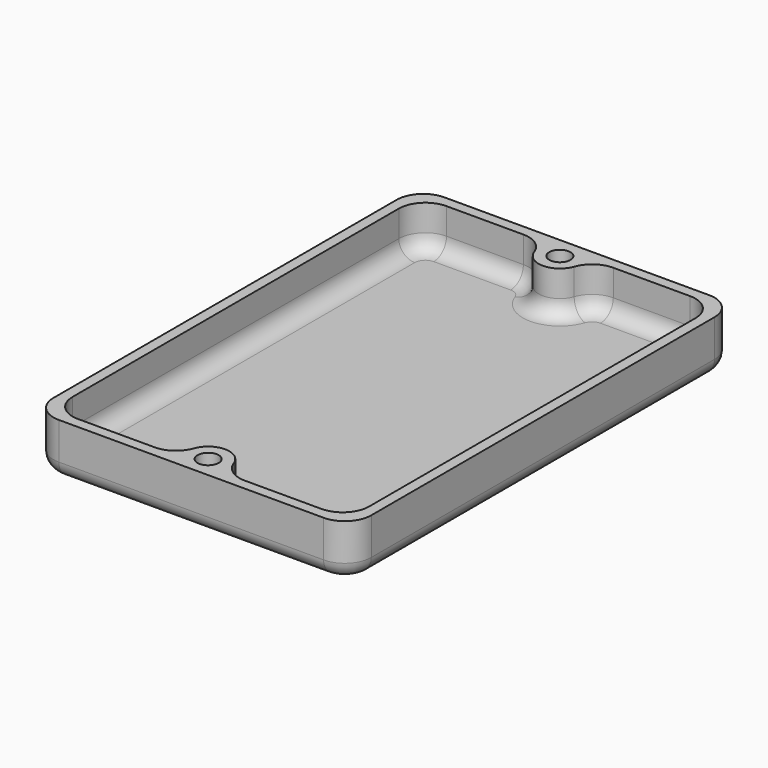
from build123d import *

# Parameters (mm, degrees)
F3_W          = 60
F3_H          = 91
F4_DEPTH      = 10
F5_W          = 56
F5_H          = 87
F6_DEPTH      = 8
F7_R          = 4
F8_DEPTH      = 10
F9_R          = 2
F10_DEPTH     = 10.001
F11_R         = 5
F12_R         = 5
F13_T1_DEPTH  = 77
F13_T3_DEPTH  = 14.5147186258
F13_T5_DEPTH  = 14.5147186258
F13_T8_ANGLE  = 90
F13_T10_ANGLE = 70.5287793655
F13_T12_ANGLE = 141.057558731
F13_T14_ANGLE = 90
F13_T16_ANGLE = 70.5287793655
F13_T18_ANGLE = 70.5287793655
F13_T20_ANGLE = 90
F13_T22_ANGLE = 141.057558731
F13_T24_ANGLE = 70.5287793655
F13_T26_ANGLE = 90
F13_T27_DEPTH = 81
F13_T29_DEPTH = 50
F13_T32_ANGLE = 90
F13_T34_ANGLE = 90
F13_T36_ANGLE = 90
F13_T38_ANGLE = 90


# Not quite as in the source:
# - a fillet or chamfer that OpenCascade refuses, or shapes differently, is made with other operations: its cross-section is extruded or revolved along the edge and cut away or added


with BuildPart() as f4:
    # F3 (on Top) → F4 (new body)
    with BuildSketch(Plane.XY):
        Rectangle(F3_W, F3_H)
    extrude(amount=F4_DEPTH)

    # F5 (on face) → F6 (cut)
    with BuildSketch(Plane.XY.offset(10)):
        Rectangle(F5_W, F5_H)
    extrude(amount=-F6_DEPTH, mode=Mode.SUBTRACT)

    # F7 (on face) → F8 (join)
    with BuildSketch(Plane(origin=(0, 0, 0), x_dir=(1, 0, 0), z_dir=(0, 0, -1))):
        with Locations((0, -41.5)):
            Circle(F7_R)
        with Locations((0, 41.5)):
            Circle(F7_R)
    extrude(amount=-F8_DEPTH)

    # F9 (on face) → F10 (cut, through all)
    with BuildSketch(Plane(origin=(0, 0, 0), x_dir=(1, 0, 0), z_dir=(0, 0, -1))):
        with Locations((0, -41.5)):
            Circle(F9_R)
        with Locations((0, 41.5)):
            Circle(F9_R)
    extrude(amount=-F10_DEPTH, mode=Mode.SUBTRACT)

    # F11
    f11_edges = [f4.edges().sort_by_distance(p)[0] for p in [
        (3.464102, 43.5, 6),
        (-3.464102, 43.5, 6),
        (-3.464102, -43.5, 6),
        (3.464102, -43.5, 6),
    ]]
    fillet(f11_edges, radius=F11_R)

    # F12
    f12_edges = [f4.edges().sort_by_distance(p)[0] for p in [
        (30, -45.5, 5),
        (-30, -45.5, 5),
        (30, 45.5, 5),
        (-30, 45.5, 5),
        (28, -43.5, 6),
        (-28, -43.5, 6),
        (-28, 43.5, 6),
        (28, 43.5, 6),
    ]]
    fillet(f12_edges, radius=F12_R)

    # F13: fillet of radius 3 on 24 edges, made by hand

    # F13_s2 → F13_t1 (join)
    with BuildSketch(Plane.XZ.offset(-38.5)):
        with BuildLine():
            ThreePointArc((-28, 5), (-27.1213203436, 2.8786796564), (-25, 2))
            Line((-25, 2), (-28, 2))
            Line((-28, 2), (-28, 5))
        make_face()
        with BuildLine():
            ThreePointArc((28, 5), (27.1213203436, 2.8786796564), (25, 2))
            Line((25, 2), (28, 2))
            Line((28, 2), (28, 5))
        make_face()
    extrude(amount=F13_T1_DEPTH)

    # F13_s4 → F13_t3 (join)
    with BuildSketch(Plane.YZ.offset(8.4852813742)):
        with BuildLine():
            ThreePointArc((-43.5, 5), (-42.6213203436, 2.8786796564), (-40.5, 2))
            Line((-40.5, 2), (-43.5, 2))
            Line((-43.5, 2), (-43.5, 5))
        make_face()
        with BuildLine():
            ThreePointArc((43.5, 5), (42.6213203436, 2.8786796564), (40.5, 2))
            Line((40.5, 2), (43.5, 2))
            Line((43.5, 2), (43.5, 5))
        make_face()
    extrude(amount=F13_T3_DEPTH)

    # F13_s6 → F13_t5 (join)
    with BuildSketch(Plane.YZ.offset(-23)):
        with BuildLine():
            ThreePointArc((-43.5, 5), (-42.6213203436, 2.8786796564), (-40.5, 2))
            Line((-40.5, 2), (-43.5, 2))
            Line((-43.5, 2), (-43.5, 5))
        make_face()
        with BuildLine():
            ThreePointArc((43.5, 5), (42.6213203436, 2.8786796564), (40.5, 2))
            Line((40.5, 2), (43.5, 2))
            Line((43.5, 2), (43.5, 5))
        make_face()
    extrude(amount=F13_T5_DEPTH)

    # F13_s7 → F13_t8 (revolve)
    with BuildSketch(Plane.YZ.offset(23)):
        with BuildLine():
            ThreePointArc((-43.5, 5), (-42.6213203436, 2.8786796564), (-40.5, 2))
            Line((-40.5, 2), (-43.5, 2))
            Line((-43.5, 2), (-43.5, 5))
        make_face()
    revolve(axis=Axis((23, -38.5, 2), (0, 0, 1)), revolution_arc=F13_T8_ANGLE)

    # F13_s9 → F13_t10 (revolve)
    with BuildSketch(Plane.YZ.offset(8.4852813742)):
        with BuildLine():
            ThreePointArc((-43.5, 5), (-42.6213203436, 2.8786796564), (-40.5, 2))
            Line((-40.5, 2), (-43.5, 2))
            Line((-43.5, 2), (-43.5, 5))
        make_face()
    revolve(axis=Axis((8.4852813742, -38.5, 2), (0, 0, -1)), revolution_arc=F13_T10_ANGLE)

    # F13_s11 → F13_t12 (revolve)
    with BuildSketch(Plane(origin=(-13.0421917419, -36.8888888889, 0), x_dir=(0, 0, 1), z_dir=(-0.3333333333, -0.9428090416, 0))):
        with BuildLine():
            ThreePointArc((5, -9.8333333333), (2.8786796564, -8.9546536769), (2, -6.8333333333))
            Line((2, -6.8333333333), (2, -9.8333333333))
            Line((2, -9.8333333333), (5, -9.8333333333))
        make_face()
    revolve(axis=Axis((0, -41.5, 2), (0, 0, -1)), revolution_arc=F13_T12_ANGLE)

    # F13_s13 → F13_t14 (revolve)
    with BuildSketch(Plane.XZ.offset(-38.5)):
        with BuildLine():
            ThreePointArc((28, 5), (27.1213203436, 2.8786796564), (25, 2))
            Line((25, 2), (28, 2))
            Line((28, 2), (28, 5))
        make_face()
    revolve(axis=Axis((23, 38.5, 2), (0, 0, 1)), revolution_arc=F13_T14_ANGLE)

    # F13_s15 → F13_t16 (revolve)
    with BuildSketch(Plane(origin=(-13.0421917419, -36.8888888889, 0), x_dir=(0, 0, 1), z_dir=(0.3333333333, 0.9428090416, 0))):
        with BuildLine():
            ThreePointArc((5, 9.8333333333), (2.8786796564, 8.9546536769), (2, 6.8333333333))
            Line((2, 6.8333333333), (2, 9.8333333333))
            Line((2, 9.8333333333), (5, 9.8333333333))
        make_face()
    revolve(axis=Axis((-8.4852813742, -38.5, 2), (0, 0, -1)), revolution_arc=F13_T16_ANGLE)

    # F13_s17 → F13_t18 (revolve)
    with BuildSketch(Plane.YZ.offset(8.4852813742)):
        with BuildLine():
            ThreePointArc((43.5, 5), (42.6213203436, 2.8786796564), (40.5, 2))
            Line((40.5, 2), (43.5, 2))
            Line((43.5, 2), (43.5, 5))
        make_face()
    revolve(axis=Axis((8.4852813742, 38.5, 2), (0, 0, 1)), revolution_arc=F13_T18_ANGLE)

    # F13_s19 → F13_t20 (revolve)
    with BuildSketch(Plane.YZ.offset(-23)):
        with BuildLine():
            ThreePointArc((-43.5, 5), (-42.6213203436, 2.8786796564), (-40.5, 2))
            Line((-40.5, 2), (-43.5, 2))
            Line((-43.5, 2), (-43.5, 5))
        make_face()
    revolve(axis=Axis((-23, -38.5, 2), (0, 0, -1)), revolution_arc=F13_T20_ANGLE)

    # F13_s21 → F13_t22 (revolve)
    with BuildSketch(Plane(origin=(13.0421917419, 36.8888888889, 0), x_dir=(0, 0, 1), z_dir=(0.3333333333, 0.9428090416, 0))):
        with BuildLine():
            ThreePointArc((5, -9.8333333333), (2.8786796564, -8.9546536769), (2, -6.8333333333))
            Line((2, -6.8333333333), (2, -9.8333333333))
            Line((2, -9.8333333333), (5, -9.8333333333))
        make_face()
    revolve(axis=Axis((0, 41.5, 2), (0, 0, -1)), revolution_arc=F13_T22_ANGLE)

    # F13_s23 → F13_t24 (revolve)
    with BuildSketch(Plane(origin=(-13.0421917419, 36.8888888889, 0), x_dir=(0, 0, 1), z_dir=(0.3333333333, -0.9428090416, 0))):
        with BuildLine():
            ThreePointArc((5, -9.8333333333), (2.8786796564, -8.9546536769), (2, -6.8333333333))
            Line((2, -6.8333333333), (2, -9.8333333333))
            Line((2, -9.8333333333), (5, -9.8333333333))
        make_face()
    revolve(axis=Axis((-8.4852813742, 38.5, 2), (0, 0, 1)), revolution_arc=F13_T24_ANGLE)

    # F13_s25 → F13_t26 (revolve)
    with BuildSketch(Plane.XZ.offset(-38.5)):
        with BuildLine():
            ThreePointArc((-28, 5), (-27.1213203436, 2.8786796564), (-25, 2))
            Line((-25, 2), (-28, 2))
            Line((-28, 2), (-28, 5))
        make_face()
    revolve(axis=Axis((-23, 38.5, 2), (0, 0, -1)), revolution_arc=F13_T26_ANGLE)

    # F13_s28 → F13_t27 (cut)
    with BuildSketch(Plane.XZ.offset(-40.5)):
        with BuildLine():
            ThreePointArc((30, 3), (29.1213203436, 0.8786796564), (27, 0))
            Line((27, 0), (30, 0))
            Line((30, 0), (30, 3))
        make_face()
        with BuildLine():
            ThreePointArc((-30, 3), (-29.1213203436, 0.8786796564), (-27, 0))
            Line((-27, 0), (-30, 0))
            Line((-30, 0), (-30, 3))
        make_face()
    extrude(amount=F13_T27_DEPTH, mode=Mode.SUBTRACT)

    # F13_s30 → F13_t29 (cut)
    with BuildSketch(Plane.YZ.offset(-25)):
        with BuildLine():
            ThreePointArc((-45.5, 3), (-44.6213203436, 0.8786796564), (-42.5, 0))
            Line((-42.5, 0), (-45.5, 0))
            Line((-45.5, 0), (-45.5, 3))
        make_face()
        with BuildLine():
            ThreePointArc((45.5, 3), (44.6213203436, 0.8786796564), (42.5, 0))
            Line((42.5, 0), (45.5, 0))
            Line((45.5, 0), (45.5, 3))
        make_face()
    extrude(amount=F13_T29_DEPTH, mode=Mode.SUBTRACT)

    # F13_s31 → F13_t32 (revolve, cut)
    with BuildSketch(Plane.YZ.offset(25)):
        with BuildLine():
            ThreePointArc((-45.5, 3), (-44.6213203436, 0.8786796564), (-42.5, 0))
            Line((-42.5, 0), (-45.5, 0))
            Line((-45.5, 0), (-45.5, 3))
        make_face()
    revolve(axis=Axis((25, -40.5, 0), (0, 0, 1)), revolution_arc=F13_T32_ANGLE, mode=Mode.SUBTRACT)

    # F13_s33 → F13_t34 (revolve, cut)
    with BuildSketch(Plane.YZ.offset(-25)):
        with BuildLine():
            ThreePointArc((-45.5, 3), (-44.6213203436, 0.8786796564), (-42.5, 0))
            Line((-42.5, 0), (-45.5, 0))
            Line((-45.5, 0), (-45.5, 3))
        make_face()
    revolve(axis=Axis((-25, -40.5, 0), (0, 0, -1)), revolution_arc=F13_T34_ANGLE, mode=Mode.SUBTRACT)

    # F13_s35 → F13_t36 (revolve, cut)
    with BuildSketch(Plane.XZ.offset(-40.5)):
        with BuildLine():
            ThreePointArc((30, 3), (29.1213203436, 0.8786796564), (27, 0))
            Line((27, 0), (30, 0))
            Line((30, 0), (30, 3))
        make_face()
    revolve(axis=Axis((25, 40.5, 0), (0, 0, 1)), revolution_arc=F13_T36_ANGLE, mode=Mode.SUBTRACT)

    # F13_s37 → F13_t38 (revolve, cut)
    with BuildSketch(Plane.XZ.offset(-40.5)):
        with BuildLine():
            ThreePointArc((-30, 3), (-29.1213203436, 0.8786796564), (-27, 0))
            Line((-27, 0), (-30, 0))
            Line((-30, 0), (-30, 3))
        make_face()
    revolve(axis=Axis((-25, 40.5, 0), (0, 0, -1)), revolution_arc=F13_T38_ANGLE, mode=Mode.SUBTRACT)


solid = f4.part
